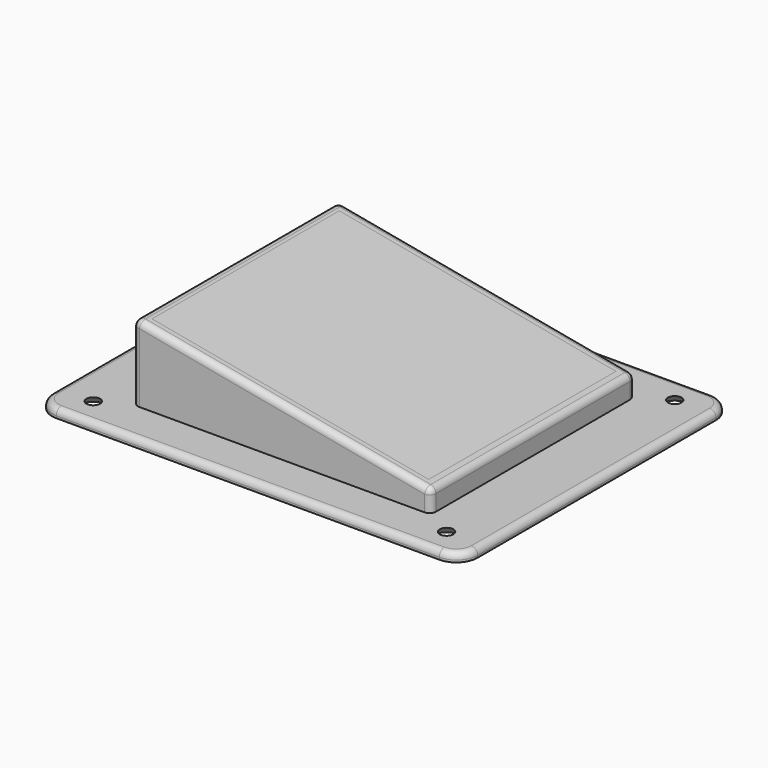
from build123d import *

# Parameters (mm, degrees)
F0_W          = 100
F0_H          = 80
F1_DEPTH      = 2
F2_W          = 70
F2_H          = 60
F3_DEPTH      = 18
F4_T          = -2.5
F6_DEPTH      = 120
F7_DEPTH      = 10
F9_W          = 71.0643865168
F9_H          = 59.9142536521
F10_DEPTH     = 2.5
F12_DEPTH     = 120
F13_R         = 1.5
F14_R         = 1.6002340802
F15_DEPTH     = 10
F16_T1_DEPTH  = 14.5
F16_T4_ANGLE  = 90
F16_T6_ANGLE  = 90
F16_T8_ANGLE  = 90
F16_T10_ANGLE = 90
F17_SIZE      = 1.99999
F18_R         = 2


# Not quite as in the source:
# - a fillet or chamfer that OpenCascade refuses, or shapes differently, is made with other operations: its cross-section is extruded or revolved along the edge and cut away or added
# - a fillet or chamfer is up to 0.001 mm smaller than in the source, because OpenCascade refuses the exact size


with BuildPart() as f1:
    # F0 (on Top) → F1 (new body)
    with BuildSketch(Plane.XY):
        Rectangle(F0_W, F0_H)
    extrude(amount=F1_DEPTH)

    # F2 (on face) → F3 (join)
    with BuildSketch(Plane.XY.offset(2)):
        Rectangle(F2_W, F2_H)
    extrude(amount=F3_DEPTH)

    # F4
    f4_openings = [f1.faces().sort_by_distance(p)[0] for p in [
        (0, 0, 20),
    ]]
    offset(amount=F4_T, openings=f4_openings)

    # F5 (on face) → F6 (cut)
    with BuildSketch(Plane.XZ.offset(30)):
        Polygon((35, 20), (-35, 20), (35, 7), align=None)
    extrude(amount=-F6_DEPTH, mode=Mode.SUBTRACT)

    # F7 (cut): a face of the model
    f7_faces = [f1.faces().sort_by_distance(p)[0] for p in [
        (0, 0, 2.5),
    ]]
    extrude(f7_faces, amount=-F7_DEPTH, mode=Mode.SUBTRACT)

    # F9 (on face) → F10 (join)
    with BuildSketch(Plane(origin=(2.4235549418, 0, 13.0499112251), x_dir=(0.9831887361, 0, -0.1825921938), z_dir=(0.1825921938, 0, 0.9831887361))):
        with Locations((-2.4766456336, 0)):
            Rectangle(F9_W, F9_H)
    extrude(amount=-F10_DEPTH)

    # F11 (on face) → F12 (cut)
    with BuildSketch(Plane.XZ.offset(29.957126826)):
        Polygon((-35, 17.4572532127), (-35, 19.7009141169), (-35.4027878127, 17.5320566636), align=None)
    extrude(amount=-F12_DEPTH, mode=Mode.SUBTRACT)

    # F13
    f13_edges = [f1.edges().sort_by_distance(p)[0] for p in [
        (0, -30, 13.5),
        (-35, 0, 20),
        (-35, -30, 11),
        (35, 0, 7),
        (35, -30, 4.5),
        (0, -40, 2),
        (50, 0, 2),
        (0, 40, 2),
        (35, 30, 4.5),
        (-35, 30, 11),
        (0, 30, 13.5),
        (-50, 0, 2),
    ]]
    fillet(f13_edges, radius=F13_R)

    # F14 (on face) → F15 (cut)
    with BuildSketch(Plane.XY.offset(2)):
        with Locations((-41.5, 33.5)):
            Circle(F14_R)
        with Locations((41.5, 33.5)):
            Circle(F14_R)
        with Locations((-41.5, -33.5)):
            Circle(F14_R)
        with Locations((41.5, -33.5)):
            Circle(F14_R)
    extrude(amount=-F15_DEPTH, mode=Mode.SUBTRACT)

    # F16: fillet of radius 5 on 4 edges, made by hand

    # F16_s2 → F16_t1 (cut)
    with BuildSketch(Plane.XY.offset(-12.5)):
        with BuildLine():
            ThreePointArc((45, -40), (48.5355339059, -38.5355339059), (50, -35))
            Line((50, -35), (50, -40))
            Line((50, -40), (45, -40))
        make_face()
        with BuildLine():
            ThreePointArc((-45, -40), (-48.5355339059, -38.5355339059), (-50, -35))
            Line((-50, -35), (-50, -40))
            Line((-50, -40), (-45, -40))
        make_face()
        with BuildLine():
            ThreePointArc((-50, 35), (-48.5355339059, 38.5355339059), (-45, 40))
            Line((-45, 40), (-50, 40))
            Line((-50, 40), (-50, 35))
        make_face()
        with BuildLine():
            ThreePointArc((50, 35), (48.5355339059, 38.5355339059), (45, 40))
            Line((45, 40), (50, 40))
            Line((50, 40), (50, 35))
        make_face()
    extrude(amount=F16_T1_DEPTH, mode=Mode.SUBTRACT)

    # F16_s3 → F16_t4 (revolve, cut)
    with BuildSketch(Plane.XZ.offset(-35)):
        with BuildLine():
            ThreePointArc((48.5, 2), (49.5606601718, 1.5606601718), (50, 0.5))
            Line((50, 0.5), (50, 2))
            Line((50, 2), (48.5, 2))
        make_face()
    revolve(axis=Axis((45, 35, 2), (0, 0, 1)), revolution_arc=F16_T4_ANGLE, mode=Mode.SUBTRACT)

    # F16_s5 → F16_t6 (revolve, cut)
    with BuildSketch(Plane.YZ.offset(-45)):
        with BuildLine():
            ThreePointArc((38.5, 2), (39.5606601718, 1.5606601718), (40, 0.5))
            Line((40, 0.5), (40, 2))
            Line((40, 2), (38.5, 2))
        make_face()
    revolve(axis=Axis((-45, 35, 2), (0, 0, 1)), revolution_arc=F16_T6_ANGLE, mode=Mode.SUBTRACT)

    # F16_s7 → F16_t8 (revolve, cut)
    with BuildSketch(Plane.XZ.offset(35)):
        with BuildLine():
            ThreePointArc((-48.5, 2), (-49.5606601718, 1.5606601718), (-50, 0.5))
            Line((-50, 0.5), (-50, 2))
            Line((-50, 2), (-48.5, 2))
        make_face()
    revolve(axis=Axis((-45, -35, 2), (0, 0, 1)), revolution_arc=F16_T8_ANGLE, mode=Mode.SUBTRACT)

    # F16_s9 → F16_t10 (revolve, cut)
    with BuildSketch(Plane.YZ.offset(45)):
        with BuildLine():
            ThreePointArc((-38.5, 2), (-39.5606601718, 1.5606601718), (-40, 0.5))
            Line((-40, 0.5), (-40, 2))
            Line((-40, 2), (-38.5, 2))
        make_face()
    revolve(axis=Axis((45, -35, 2), (0, 0, 1)), revolution_arc=F16_T10_ANGLE, mode=Mode.SUBTRACT)

    # F17 (size 2 in the source; OpenCascade refuses exactly that, so slightly less here)
    f17_edges = [f1.edges().sort_by_distance(p)[0] for p in [
        (39.899766, -33.5, 0),
        (39.899766, 33.5, 0),
        (-43.100234, -33.5, 0),
        (-43.100234, 33.5, 0),
    ]]
    chamfer(f17_edges, length=F17_SIZE)

    # F18
    f18_edges = [f1.edges().sort_by_distance(p)[0] for p in [
        (32.5, 0, 0),
        (0, -27.5, 0),
        (0, 27.5, 0),
        (-32.5, 0, 0),
    ]]
    fillet(f18_edges, radius=F18_R)


solid = f1.part
